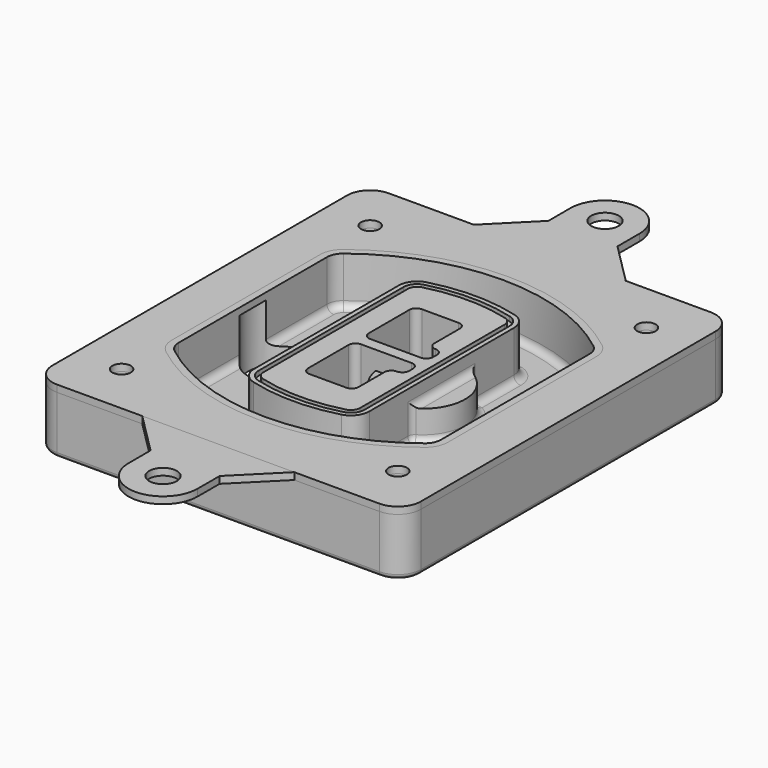
from build123d import *

# Parameters (mm, degrees)
F0_R      = 4
F1_DEPTH  = 25
F2_DEPTH  = 3
F3_DEPTH  = 18
F5_DEPTH  = 21
F6_DEPTH  = 2
F8_DEPTH  = 20
F9_DEPTH  = 16
F10_DEPTH = 25
F7_R      = 6
F7_R_2    = 4
F11_DEPTH = 6
F13_DEPTH = 9
F14_R     = 3
F15_R     = 2
F16_R     = 6
F16_R_2   = 4
F17_DEPTH = 3
F18_DEPTH = 3


# Not quite as in the source:
# - a feature names something its author has since deleted; it is built from what else it names


with BuildPart() as f1:
    # F0 (on Top) → F1 (new body)
    with BuildSketch(Plane.XY):
        with BuildLine():
            ThreePointArc((-80, -80), (-77.0710678119, -87.0710678119), (-70, -90))
            Line((-70, -90), (70, -90))
            ThreePointArc((70, -90), (77.0710678119, -87.0710678119), (80, -80))
            Line((80, -80), (80, 80))
            ThreePointArc((80, 80), (77.0710678119, 87.0710678119), (70, 90))
            Line((70, 90), (-70, 90))
            ThreePointArc((-70, 90), (-77.0710678119, 87.0710678119), (-80, 80))
            Line((-80, 80), (-80, -80))
        make_face()
        with Locations((-60, -67.5)):
            Circle(F0_R, mode=Mode.SUBTRACT)
        with Locations((60, -67.5)):
            Circle(F0_R, mode=Mode.SUBTRACT)
        with Locations((-60, 67.5)):
            Circle(F0_R, mode=Mode.SUBTRACT)
        with BuildLine():
            ThreePointArc((-64, 40.2934422872), (-62.5820384798, 46.4328484224), (-58.6153846154, 51.3286200352))
            ThreePointArc((-58.6153846154, 51.3286200352), (0, 71.5), (58.6153846154, 51.3286200352))
            ThreePointArc((58.6153846154, 51.3286200352), (62.5820384798, 46.4328484224), (64, 40.2934422872))
            Line((64, 40.2934422872), (64, -40.2934422872))
            ThreePointArc((64, -40.2934422872), (62.5820384798, -46.4328484224), (58.6153846154, -51.3286200352))
            ThreePointArc((58.6153846154, -51.3286200352), (0, -71.5), (-58.6153846154, -51.3286200352))
            ThreePointArc((-58.6153846154, -51.3286200352), (-62.5820384798, -46.4328484224), (-64, -40.2934422872))
            Line((-64, -40.2934422872), (-64, 40.2934422872))
        make_face(mode=Mode.SUBTRACT)
        with Locations((60, 67.5)):
            Circle(F0_R, mode=Mode.SUBTRACT)
        with BuildLine():
            ThreePointArc((58.6153846154, 51.3286200352), (0, 71.5), (-58.6153846154, 51.3286200352))
            ThreePointArc((-58.6153846154, 51.3286200352), (-62.5820384798, 46.4328484224), (-64, 40.2934422872))
            Line((-64, 40.2934422872), (-64, -40.2934422872))
            ThreePointArc((-64, -40.2934422872), (-62.5820384798, -46.4328484224), (-58.6153846154, -51.3286200352))
            ThreePointArc((-58.6153846154, -51.3286200352), (0, -71.5), (58.6153846154, -51.3286200352))
            ThreePointArc((58.6153846154, -51.3286200352), (62.5820384798, -46.4328484224), (64, -40.2934422872))
            Line((64, -40.2934422872), (64, 40.2934422872))
            ThreePointArc((64, 40.2934422872), (62.5820384798, 46.4328484224), (58.6153846154, 51.3286200352))
        make_face()
        with BuildLine():
            Line((-60, -40.2934422872), (-60, 40.2934422872))
            ThreePointArc((-60, 40.2934422872), (-58.9871703427, 44.6787323838), (-56.1538461538, 48.1757121072))
            ThreePointArc((-56.1538461538, 48.1757121072), (0, 67.5), (56.1538461538, 48.1757121072))
            ThreePointArc((56.1538461538, 48.1757121072), (58.9871703427, 44.6787323838), (60, 40.2934422872))
            Line((60, 40.2934422872), (60, -40.2934422872))
            ThreePointArc((60, -40.2934422872), (58.9871703427, -44.6787323838), (56.1538461538, -48.1757121072))
            ThreePointArc((56.1538461538, -48.1757121072), (0, -67.5), (-56.1538461538, -48.1757121072))
            ThreePointArc((-56.1538461538, -48.1757121072), (-58.9871703427, -44.6787323838), (-60, -40.2934422872))
        make_face(mode=Mode.SUBTRACT)
        with BuildLine():
            ThreePointArc((-56.1538461538, 48.1757121072), (-58.9871703427, 44.6787323838), (-60, 40.2934422872))
            Line((-60, 40.2934422872), (-60, -40.2934422872))
            ThreePointArc((-60, -40.2934422872), (-58.9871703427, -44.6787323838), (-56.1538461538, -48.1757121072))
            ThreePointArc((-56.1538461538, -48.1757121072), (0, -67.5), (56.1538461538, -48.1757121072))
            ThreePointArc((56.1538461538, -48.1757121072), (58.9871703427, -44.6787323838), (60, -40.2934422872))
            Line((60, -40.2934422872), (60, 40.2934422872))
            ThreePointArc((60, 40.2934422872), (58.9871703427, 44.6787323838), (56.1538461538, 48.1757121072))
            ThreePointArc((56.1538461538, 48.1757121072), (0, 67.5), (-56.1538461538, 48.1757121072))
        make_face()
        with BuildLine():
            ThreePointArc((54.3076923077, 45.8110311612), (56.2910192399, 43.3631453548), (57, 40.2934422872))
            Line((57, 40.2934422872), (57, -40.2934422872))
            ThreePointArc((57, -40.2934422872), (56.2910192399, -43.3631453548), (54.3076923077, -45.8110311612))
            ThreePointArc((54.3076923077, -45.8110311612), (0, -64.5), (-54.3076923077, -45.8110311612))
            ThreePointArc((-54.3076923077, -45.8110311612), (-56.2910192399, -43.3631453548), (-57, -40.2934422872))
            Line((-57, -40.2934422872), (-57, 40.2934422872))
            ThreePointArc((-57, 40.2934422872), (-56.2910192399, 43.3631453548), (-54.3076923077, 45.8110311612))
            ThreePointArc((-54.3076923077, 45.8110311612), (0, 64.5), (54.3076923077, 45.8110311612))
        make_face(mode=Mode.SUBTRACT)
        with BuildLine():
            Line((57, -40.2934422872), (57, 40.2934422872))
            ThreePointArc((57, 40.2934422872), (56.2910192399, 43.3631453548), (54.3076923077, 45.8110311612))
            ThreePointArc((54.3076923077, 45.8110311612), (0, 64.5), (-54.3076923077, 45.8110311612))
            ThreePointArc((-54.3076923077, 45.8110311612), (-56.2910192399, 43.3631453548), (-57, 40.2934422872))
            Line((-57, 40.2934422872), (-57, -40.2934422872))
            ThreePointArc((-57, -40.2934422872), (-56.2910192399, -43.3631453548), (-54.3076923077, -45.8110311612))
            ThreePointArc((-54.3076923077, -45.8110311612), (0, -64.5), (54.3076923077, -45.8110311612))
            ThreePointArc((54.3076923077, -45.8110311612), (56.2910192399, -43.3631453548), (57, -40.2934422872))
        make_face()
    extrude(amount=-F1_DEPTH)

    # F0 (on Top) → F2 (join)
    with BuildSketch(Plane.XY):
        with BuildLine():
            ThreePointArc((-56.1538461538, 48.1757121072), (-58.9871703427, 44.6787323838), (-60, 40.2934422872))
            Line((-60, 40.2934422872), (-60, -40.2934422872))
            ThreePointArc((-60, -40.2934422872), (-58.9871703427, -44.6787323838), (-56.1538461538, -48.1757121072))
            ThreePointArc((-56.1538461538, -48.1757121072), (0, -67.5), (56.1538461538, -48.1757121072))
            ThreePointArc((56.1538461538, -48.1757121072), (58.9871703427, -44.6787323838), (60, -40.2934422872))
            Line((60, -40.2934422872), (60, 40.2934422872))
            ThreePointArc((60, 40.2934422872), (58.9871703427, 44.6787323838), (56.1538461538, 48.1757121072))
            ThreePointArc((56.1538461538, 48.1757121072), (0, 67.5), (-56.1538461538, 48.1757121072))
        make_face()
        with BuildLine():
            ThreePointArc((54.3076923077, 45.8110311612), (56.2910192399, 43.3631453548), (57, 40.2934422872))
            Line((57, 40.2934422872), (57, -40.2934422872))
            ThreePointArc((57, -40.2934422872), (56.2910192399, -43.3631453548), (54.3076923077, -45.8110311612))
            ThreePointArc((54.3076923077, -45.8110311612), (0, -64.5), (-54.3076923077, -45.8110311612))
            ThreePointArc((-54.3076923077, -45.8110311612), (-56.2910192399, -43.3631453548), (-57, -40.2934422872))
            Line((-57, -40.2934422872), (-57, 40.2934422872))
            ThreePointArc((-57, 40.2934422872), (-56.2910192399, 43.3631453548), (-54.3076923077, 45.8110311612))
            ThreePointArc((-54.3076923077, 45.8110311612), (0, 64.5), (54.3076923077, 45.8110311612))
        make_face(mode=Mode.SUBTRACT)
    extrude(amount=F2_DEPTH)

    # F0 (on Top) → F3 (cut)
    with BuildSketch(Plane.XY):
        with BuildLine():
            Line((57, -40.2934422872), (57, 40.2934422872))
            ThreePointArc((57, 40.2934422872), (56.2910192399, 43.3631453548), (54.3076923077, 45.8110311612))
            ThreePointArc((54.3076923077, 45.8110311612), (0, 64.5), (-54.3076923077, 45.8110311612))
            ThreePointArc((-54.3076923077, 45.8110311612), (-56.2910192399, 43.3631453548), (-57, 40.2934422872))
            Line((-57, 40.2934422872), (-57, -40.2934422872))
            ThreePointArc((-57, -40.2934422872), (-56.2910192399, -43.3631453548), (-54.3076923077, -45.8110311612))
            ThreePointArc((-54.3076923077, -45.8110311612), (0, -64.5), (54.3076923077, -45.8110311612))
            ThreePointArc((54.3076923077, -45.8110311612), (56.2910192399, -43.3631453548), (57, -40.2934422872))
        make_face()
    extrude(amount=-F3_DEPTH, mode=Mode.SUBTRACT)

    # F4 (on face) → F5 (join, through all)
    with BuildSketch(Plane.XY.offset(3)):
        with BuildLine():
            ThreePointArc((-25, -39.2465276821), (-23.3511545998, -44.1109737193), (-19.0842911877, -46.9702398883))
            ThreePointArc((-19.0842911877, -46.9702398883), (0, -49.5), (19.0842911877, -46.9702398883))
            ThreePointArc((19.0842911877, -46.9702398883), (23.3511545998, -44.1109737193), (25, -39.2465276821))
            Line((25, -39.2465276821), (25, 39.2465276821))
            ThreePointArc((25, 39.2465276821), (23.3511545998, 44.1109737193), (19.0842911877, 46.9702398883))
            ThreePointArc((19.0842911877, 46.9702398883), (0, 49.5), (-19.0842911877, 46.9702398883))
            ThreePointArc((-19.0842911877, 46.9702398883), (-23.3511545998, 44.1109737193), (-25, 39.2465276821))
            Line((-25, 39.2465276821), (-25, -39.2465276821))
        make_face()
        with BuildLine():
            ThreePointArc((18.5632183908, 45.0393118368), (21.7633659499, 42.89486221), (23, 39.2465276821))
            Line((23, 39.2465276821), (23, -39.2465276821))
            ThreePointArc((23, -39.2465276821), (21.7633659499, -42.89486221), (18.5632183908, -45.0393118368))
            ThreePointArc((18.5632183908, -45.0393118368), (0, -47.5), (-18.5632183908, -45.0393118368))
            ThreePointArc((-18.5632183908, -45.0393118368), (-21.7633659499, -42.89486221), (-23, -39.2465276821))
            Line((-23, -39.2465276821), (-23, 39.2465276821))
            ThreePointArc((-23, 39.2465276821), (-21.7633659499, 42.89486221), (-18.5632183908, 45.0393118368))
            ThreePointArc((-18.5632183908, 45.0393118368), (0, 47.5), (18.5632183908, 45.0393118368))
        make_face(mode=Mode.SUBTRACT)
        with BuildLine():
            Line((23, -39.2465276821), (23, 39.2465276821))
            ThreePointArc((23, 39.2465276821), (21.7633659499, 42.89486221), (18.5632183908, 45.0393118368))
            ThreePointArc((18.5632183908, 45.0393118368), (0, 47.5), (-18.5632183908, 45.0393118368))
            ThreePointArc((-18.5632183908, 45.0393118368), (-21.7633659499, 42.89486221), (-23, 39.2465276821))
            Line((-23, 39.2465276821), (-23, -39.2465276821))
            ThreePointArc((-23, -39.2465276821), (-21.7633659499, -42.89486221), (-18.5632183908, -45.0393118368))
            ThreePointArc((-18.5632183908, -45.0393118368), (0, -47.5), (18.5632183908, -45.0393118368))
            ThreePointArc((18.5632183908, -45.0393118368), (21.7633659499, -42.89486221), (23, -39.2465276821))
        make_face()
        with BuildLine():
            ThreePointArc((18.0421455939, 43.1083837852), (20.1755772999, 41.6787507007), (21, 39.2465276821))
            Line((21, 39.2465276821), (21, -39.2465276821))
            ThreePointArc((21, -39.2465276821), (20.1755772999, -41.6787507007), (18.0421455939, -43.1083837852))
            ThreePointArc((18.0421455939, -43.1083837852), (0, -45.5), (-18.0421455939, -43.1083837852))
            ThreePointArc((-18.0421455939, -43.1083837852), (-20.1755772999, -41.6787507007), (-21, -39.2465276821))
            Line((-21, -39.2465276821), (-21, 39.2465276821))
            ThreePointArc((-21, 39.2465276821), (-20.1755772999, 41.6787507007), (-18.0421455939, 43.1083837852))
            ThreePointArc((-18.0421455939, 43.1083837852), (0, 45.5), (18.0421455939, 43.1083837852))
        make_face(mode=Mode.SUBTRACT)
        with BuildLine():
            Line((21, -39.2465276821), (21, 39.2465276821))
            ThreePointArc((21, 39.2465276821), (20.1755772999, 41.6787507007), (18.0421455939, 43.1083837852))
            ThreePointArc((18.0421455939, 43.1083837852), (0, 45.5), (-18.0421455939, 43.1083837852))
            ThreePointArc((-18.0421455939, 43.1083837852), (-20.1755772999, 41.6787507007), (-21, 39.2465276821))
            Line((-21, 39.2465276821), (-21, -39.2465276821))
            ThreePointArc((-21, -39.2465276821), (-20.1755772999, -41.6787507007), (-18.0421455939, -43.1083837852))
            ThreePointArc((-18.0421455939, -43.1083837852), (0, -45.5), (18.0421455939, -43.1083837852))
            ThreePointArc((18.0421455939, -43.1083837852), (20.1755772999, -41.6787507007), (21, -39.2465276821))
        make_face()
        with BuildLine():
            Line((-8, -2.5), (14, -2.5))
            ThreePointArc((14, -2.5), (16.1213203436, -3.3786796564), (17, -5.5))
            Line((17, -5.5), (17, -7.5))
            ThreePointArc((17, -7.5), (16.1213203436, -9.6213203436), (14, -10.5))
            ThreePointArc((14, -10.5), (11.8786796564, -11.3786796564), (11, -13.5))
            Line((11, -13.5), (11, -27.5))
            ThreePointArc((11, -27.5), (10.1213203436, -29.6213203436), (8, -30.5))
            Line((8, -30.5), (-8, -30.5))
            ThreePointArc((-8, -30.5), (-10.1213203436, -29.6213203436), (-11, -27.5))
            Line((-11, -27.5), (-11, -5.5))
            ThreePointArc((-11, -5.5), (-10.1213203436, -3.3786796564), (-8, -2.5))
        make_face(mode=Mode.SUBTRACT)
        with BuildLine():
            ThreePointArc((-8, 2.5), (-10.1213203436, 3.3786796564), (-11, 5.5))
            Line((-11, 5.5), (-11, 27.5))
            ThreePointArc((-11, 27.5), (-10.1213203436, 29.6213203436), (-8, 30.5))
            Line((-8, 30.5), (8, 30.5))
            ThreePointArc((8, 30.5), (10.1213203436, 29.6213203436), (11, 27.5))
            Line((11, 27.5), (11, 13.5))
            ThreePointArc((11, 13.5), (11.8786796564, 11.3786796564), (14, 10.5))
            ThreePointArc((14, 10.5), (16.1213203436, 9.6213203436), (17, 7.5))
            Line((17, 7.5), (17, 5.5))
            ThreePointArc((17, 5.5), (16.1213203436, 3.3786796564), (14, 2.5))
            Line((14, 2.5), (-8, 2.5))
        make_face(mode=Mode.SUBTRACT)
    extrude(amount=-F5_DEPTH)

    # F4 (on face) → F6 (cut)
    with BuildSketch(Plane.XY.offset(3)):
        with BuildLine():
            Line((23, -39.2465276821), (23, 39.2465276821))
            ThreePointArc((23, 39.2465276821), (21.7633659499, 42.89486221), (18.5632183908, 45.0393118368))
            ThreePointArc((18.5632183908, 45.0393118368), (0, 47.5), (-18.5632183908, 45.0393118368))
            ThreePointArc((-18.5632183908, 45.0393118368), (-21.7633659499, 42.89486221), (-23, 39.2465276821))
            Line((-23, 39.2465276821), (-23, -39.2465276821))
            ThreePointArc((-23, -39.2465276821), (-21.7633659499, -42.89486221), (-18.5632183908, -45.0393118368))
            ThreePointArc((-18.5632183908, -45.0393118368), (0, -47.5), (18.5632183908, -45.0393118368))
            ThreePointArc((18.5632183908, -45.0393118368), (21.7633659499, -42.89486221), (23, -39.2465276821))
        make_face()
        with BuildLine():
            ThreePointArc((18.0421455939, 43.1083837852), (20.1755772999, 41.6787507007), (21, 39.2465276821))
            Line((21, 39.2465276821), (21, -39.2465276821))
            ThreePointArc((21, -39.2465276821), (20.1755772999, -41.6787507007), (18.0421455939, -43.1083837852))
            ThreePointArc((18.0421455939, -43.1083837852), (0, -45.5), (-18.0421455939, -43.1083837852))
            ThreePointArc((-18.0421455939, -43.1083837852), (-20.1755772999, -41.6787507007), (-21, -39.2465276821))
            Line((-21, -39.2465276821), (-21, 39.2465276821))
            ThreePointArc((-21, 39.2465276821), (-20.1755772999, 41.6787507007), (-18.0421455939, 43.1083837852))
            ThreePointArc((-18.0421455939, 43.1083837852), (0, 45.5), (18.0421455939, 43.1083837852))
        make_face(mode=Mode.SUBTRACT)
    extrude(amount=-F6_DEPTH, mode=Mode.SUBTRACT)

    # F7 (on face) → F8 (join)
    with BuildSketch(Plane(origin=(0, 0, -25), x_dir=(1, 0, 0), z_dir=(0, 0, -1))):
        with BuildLine():
            ThreePointArc((3.28842436, 0), (16.7567035675, 13.4682792075), (30.224982775, 0))
            Line((30.224982775, 0), (35.224982775, 0))
            ThreePointArc((35.224982775, 0), (16.7567035675, 18.4682792075), (-1.71157564, 0))
            Line((-1.71157564, 0), (3.28842436, 0))
        make_face()
        with BuildLine():
            Line((3.28842436, 0), (30.224982775, 0))
            ThreePointArc((30.224982775, 0), (16.7567035675, 13.4682792075), (3.28842436, 0))
        make_face()
        with BuildLine():
            ThreePointArc((3.28842436, 0), (16.7567035675, -13.4682792075), (30.224982775, 0))
            Line((30.224982775, 0), (3.28842436, 0))
        make_face()
        with BuildLine():
            Line((35.224982775, 0), (30.224982775, 0))
            ThreePointArc((30.224982775, 0), (16.7567035675, -13.4682792075), (3.28842436, 0))
            Line((3.28842436, 0), (-1.71157564, 0))
            ThreePointArc((-1.71157564, 0), (16.7567035675, -18.4682792075), (35.224982775, 0))
        make_face()
    extrude(amount=-F8_DEPTH)

    # F7 (on face) → F9 (cut)
    with BuildSketch(Plane(origin=(0, 0, -25), x_dir=(1, 0, 0), z_dir=(0, 0, -1))):
        with BuildLine():
            Line((3.28842436, 0), (30.224982775, 0))
            ThreePointArc((30.224982775, 0), (16.7567035675, 13.4682792075), (3.28842436, 0))
        make_face()
        with BuildLine():
            ThreePointArc((3.28842436, 0), (16.7567035675, -13.4682792075), (30.224982775, 0))
            Line((30.224982775, 0), (3.28842436, 0))
        make_face()
    extrude(amount=-F9_DEPTH, mode=Mode.SUBTRACT)

    # F7 (on face) → F10 (cut)
    with BuildSketch(Plane(origin=(0, 0, -25), x_dir=(1, 0, 0), z_dir=(0, 0, -1))):
        with BuildLine():
            Line((-59.0318229325, 0), (-32.0952645175, 0))
            ThreePointArc((-32.0952645175, 0), (-45.563543725, 13.4682792075), (-59.0318229325, 0))
        make_face()
        with BuildLine():
            ThreePointArc((-59.0318229325, 0), (-45.563543725, -13.4682792075), (-32.0952645175, 0))
            Line((-32.0952645175, 0), (-59.0318229325, 0))
        make_face()
    extrude(amount=-F10_DEPTH, mode=Mode.SUBTRACT)

    # F7 (on face) → F11 (cut)
    with BuildSketch(Plane(origin=(0, 0, -25), x_dir=(1, 0, 0), z_dir=(0, 0, -1))):
        with Locations((60, -67.5)):
            Circle(F7_R)
        with Locations((60, -67.5)):
            Circle(F7_R_2, mode=Mode.SUBTRACT)
        with Locations((-60, -67.5)):
            Circle(F7_R)
        with Locations((-60, -67.5)):
            Circle(F7_R_2, mode=Mode.SUBTRACT)
        with Locations((-60, 67.5)):
            Circle(F7_R)
        with Locations((-60, 67.5)):
            Circle(F7_R_2, mode=Mode.SUBTRACT)
        with Locations((60, 67.5)):
            Circle(F7_R)
        with Locations((60, 67.5)):
            Circle(F7_R_2, mode=Mode.SUBTRACT)
    extrude(amount=-F11_DEPTH, mode=Mode.SUBTRACT)

    # F12 (on face) → F13 (cut, through all)
    with BuildSketch(Plane(origin=(0, 0, -9), x_dir=(1, 0, 0), z_dir=(0, 0, -1))):
        with BuildLine():
            Line((11, 13.5), (11, 17.5481537753))
            ThreePointArc((11, 17.5481537753), (2.5696536419, 11.8239143813), (-1.5415842455, 2.5))
            Line((-1.5415842455, 2.5), (3.5224848595, 2.5))
            ThreePointArc((3.5224848595, 2.5), (6.1857188154, 8.3455872281), (11.2536447004, 12.2927168648))
            ThreePointArc((11.2536447004, 12.2927168648), (11.0640958889, 12.8831798879), (11, 13.5))
        make_face()
        with BuildLine():
            ThreePointArc((11.2536447004, -12.2927168648), (6.1857188154, -8.3455872281), (3.5224848595, -2.5))
            Line((3.5224848595, -2.5), (-1.5415842455, -2.5))
            ThreePointArc((-1.5415842455, -2.5), (2.5696536419, -11.8239143813), (11, -17.5481537753))
            Line((11, -17.5481537753), (11, -13.5))
            ThreePointArc((11, -13.5), (11.0640958889, -12.8831798879), (11.2536447004, -12.2927168648))
        make_face()
        with BuildLine():
            ThreePointArc((11.2536447004, 12.2927168648), (6.1857188154, 8.3455872281), (3.5224848595, 2.5))
            Line((3.5224848595, 2.5), (14, 2.5))
            ThreePointArc((14, 2.5), (16.1213203436, 3.3786796564), (17, 5.5))
            Line((17, 5.5), (17, 7.5))
            ThreePointArc((17, 7.5), (16.1213203436, 9.6213203436), (14, 10.5))
            ThreePointArc((14, 10.5), (12.3601599782, 10.9878446101), (11.2536447004, 12.2927168648))
        make_face()
        with BuildLine():
            Line((14, -2.5), (3.5224848595, -2.5))
            ThreePointArc((3.5224848595, -2.5), (6.1857188154, -8.3455872281), (11.2536447004, -12.2927168648))
            ThreePointArc((11.2536447004, -12.2927168648), (12.3601599782, -10.9878446101), (14, -10.5))
            ThreePointArc((14, -10.5), (16.1213203436, -9.6213203436), (17, -7.5))
            Line((17, -7.5), (17, -5.5))
            ThreePointArc((17, -5.5), (16.1213203436, -3.3786796564), (14, -2.5))
        make_face()
    extrude(amount=F13_DEPTH, mode=Mode.SUBTRACT)

    # F14
    f14_edges = [f1.edges().sort_by_distance(p)[0] for p in [
        (-57, -23.703476, -18),
        (-57, 23.703476, -18),
        (25, 0, -5),
        (25, 16.526506, -11.5),
        (25, -16.526506, -11.5),
        (25, -27.886517, -18),
        (35.224983, 0, -18),
    ]]
    fillet(f14_edges, radius=F14_R)

    # F15
    f15_edges = [f1.edges().sort_by_distance(p)[0] for p in [
        (0, -90, -25),
    ]]
    fillet(f15_edges, radius=F15_R)


with BuildPart() as f17:
    # F16 (on face) → F17 (new body, through all)
    with BuildSketch(Plane.XY):
        with BuildLine():
            Line((15.0149209161, 108.0000092764), (15, 120))
            ThreePointArc((15, 120), (0, 134.9813604359), (-15, 120))
            Line((-15, 120), (-15, 108))
            Line((-15, 108), (-33, 90))
            Line((-33, 90), (33.0149301925, 90))
            Line((33.0149301925, 90), (15.0149209161, 108.0000092764))
        make_face()
        with Locations((0, 120)):
            Circle(F16_R, mode=Mode.SUBTRACT)
        with BuildLine():
            Line((15.0149209161, -108.0000092764), (33.0149301925, -90))
            Line((33.0149301925, -90), (-33, -90))
            Line((-33, -90), (-15, -108))
            Line((-15, -108), (-15, -120))
            ThreePointArc((-15, -120), (0, -134.9813604359), (15, -120))
            Line((15, -120), (15.0149209161, -108.0000092764))
        make_face()
        with Locations((0, -120)):
            Circle(F16_R, mode=Mode.SUBTRACT)
        with BuildLine():
            Line((70, 90), (33.0149301925, 90))
            Line((33.0149301925, 90), (-33, 90))
            Line((-33, 90), (-70, 90))
            ThreePointArc((-70, 90), (-77.0710678119, 87.0710678119), (-80, 80))
            Line((-80, 80), (-80, -80))
            ThreePointArc((-80, -80), (-77.0710678119, -87.0710678119), (-70, -90))
            Line((-70, -90), (-33, -90))
            Line((-33, -90), (33.0149301925, -90))
            Line((33.0149301925, -90), (70, -90))
            ThreePointArc((70, -90), (77.0710678119, -87.0710678119), (80, -80))
            Line((80, -80), (80, 80))
            ThreePointArc((80, 80), (77.0710678119, 87.0710678119), (70, 90))
        make_face()
        with Locations((-60, -67.5)):
            Circle(F16_R_2, mode=Mode.SUBTRACT)
        with Locations((60, -67.5)):
            Circle(F16_R_2, mode=Mode.SUBTRACT)
        with Locations((-60, 67.5)):
            Circle(F16_R_2, mode=Mode.SUBTRACT)
        with BuildLine():
            ThreePointArc((-60, 40.2934422872), (-58.9871703427, 44.6787323838), (-56.1538461538, 48.1757121072))
            ThreePointArc((-56.1538461538, 48.1757121072), (0, 67.5), (56.1538461538, 48.1757121072))
            ThreePointArc((56.1538461538, 48.1757121072), (58.9871703427, 44.6787323838), (60, 40.2934422872))
            Line((60, 40.2934422872), (60, -40.2934422872))
            ThreePointArc((60, -40.2934422872), (58.9871703427, -44.6787323838), (56.1538461538, -48.1757121072))
            ThreePointArc((56.1538461538, -48.1757121072), (0, -67.5), (-56.1538461538, -48.1757121072))
            ThreePointArc((-56.1538461538, -48.1757121072), (-58.9871703427, -44.6787323838), (-60, -40.2934422872))
            Line((-60, -40.2934422872), (-60, 40.2934422872))
        make_face(mode=Mode.SUBTRACT)
        with Locations((60, 67.5)):
            Circle(F16_R_2, mode=Mode.SUBTRACT)
    extrude(amount=F17_DEPTH)


with BuildPart() as f18:
    # F16 (on face) → F18 (new body, through all)
    with BuildSketch(Plane.XY):
        with BuildLine():
            Line((15.0149209161, 108.0000092764), (15, 120))
            ThreePointArc((15, 120), (0, 134.9813604359), (-15, 120))
            Line((-15, 120), (-15, 108))
            Line((-15, 108), (-33, 90))
            Line((-33, 90), (33.0149301925, 90))
            Line((33.0149301925, 90), (15.0149209161, 108.0000092764))
        make_face()
        with Locations((0, 120)):
            Circle(F16_R, mode=Mode.SUBTRACT)
        with BuildLine():
            Line((70, 90), (33.0149301925, 90))
            Line((33.0149301925, 90), (-33, 90))
            Line((-33, 90), (-70, 90))
            ThreePointArc((-70, 90), (-77.0710678119, 87.0710678119), (-80, 80))
            Line((-80, 80), (-80, -80))
            ThreePointArc((-80, -80), (-77.0710678119, -87.0710678119), (-70, -90))
            Line((-70, -90), (-33, -90))
            Line((-33, -90), (33.0149301925, -90))
            Line((33.0149301925, -90), (70, -90))
            ThreePointArc((70, -90), (77.0710678119, -87.0710678119), (80, -80))
            Line((80, -80), (80, 80))
            ThreePointArc((80, 80), (77.0710678119, 87.0710678119), (70, 90))
        make_face()
        with Locations((-60, -67.5)):
            Circle(F16_R_2, mode=Mode.SUBTRACT)
        with Locations((60, -67.5)):
            Circle(F16_R_2, mode=Mode.SUBTRACT)
        with Locations((-60, 67.5)):
            Circle(F16_R_2, mode=Mode.SUBTRACT)
        with BuildLine():
            ThreePointArc((-60, 40.2934422872), (-58.9871703427, 44.6787323838), (-56.1538461538, 48.1757121072))
            ThreePointArc((-56.1538461538, 48.1757121072), (0, 67.5), (56.1538461538, 48.1757121072))
            ThreePointArc((56.1538461538, 48.1757121072), (58.9871703427, 44.6787323838), (60, 40.2934422872))
            Line((60, 40.2934422872), (60, -40.2934422872))
            ThreePointArc((60, -40.2934422872), (58.9871703427, -44.6787323838), (56.1538461538, -48.1757121072))
            ThreePointArc((56.1538461538, -48.1757121072), (0, -67.5), (-56.1538461538, -48.1757121072))
            ThreePointArc((-56.1538461538, -48.1757121072), (-58.9871703427, -44.6787323838), (-60, -40.2934422872))
            Line((-60, -40.2934422872), (-60, 40.2934422872))
        make_face(mode=Mode.SUBTRACT)
        with Locations((60, 67.5)):
            Circle(F16_R_2, mode=Mode.SUBTRACT)
    extrude(amount=F18_DEPTH)


solid = Compound([f1.part, f17.part, f18.part])
